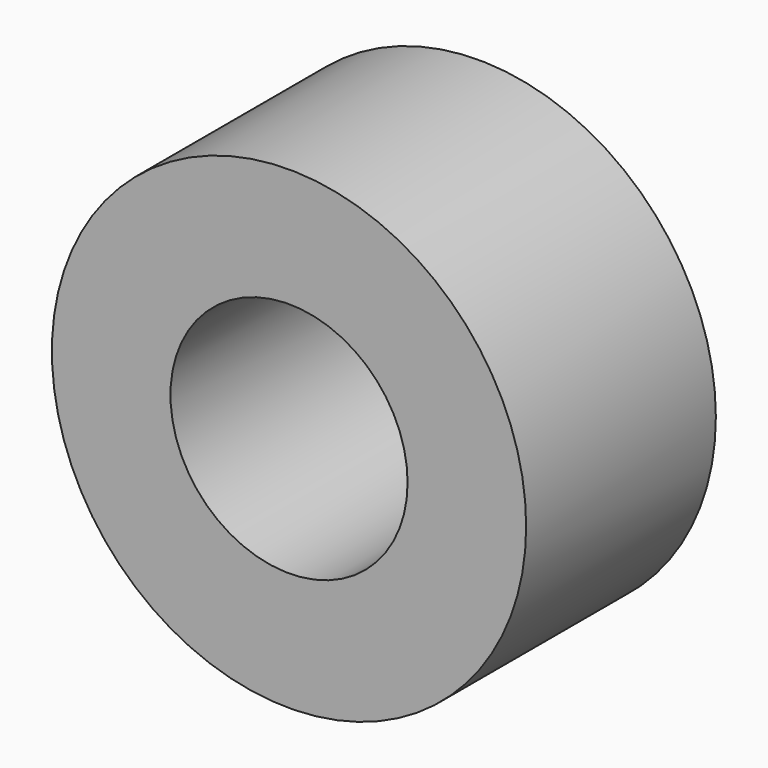
from build123d import *

# Parameters (mm, degrees)
F0_R     = 3.175
F0_R_2   = 1.5875
F1_DEPTH = 3.175


# Not quite as in the source:
# - a length typed as a fraction of an inch, garbled in the dataset ("3 / 203.2 mm" for 3/8 in), is restored


with BuildPart() as f1:
    # F0 (on Front) → F1 (new body)
    with BuildSketch(Plane.XZ):
        Circle(F0_R)
        Circle(F0_R_2, mode=Mode.SUBTRACT)
    extrude(amount=F1_DEPTH)


solid = f1.part
